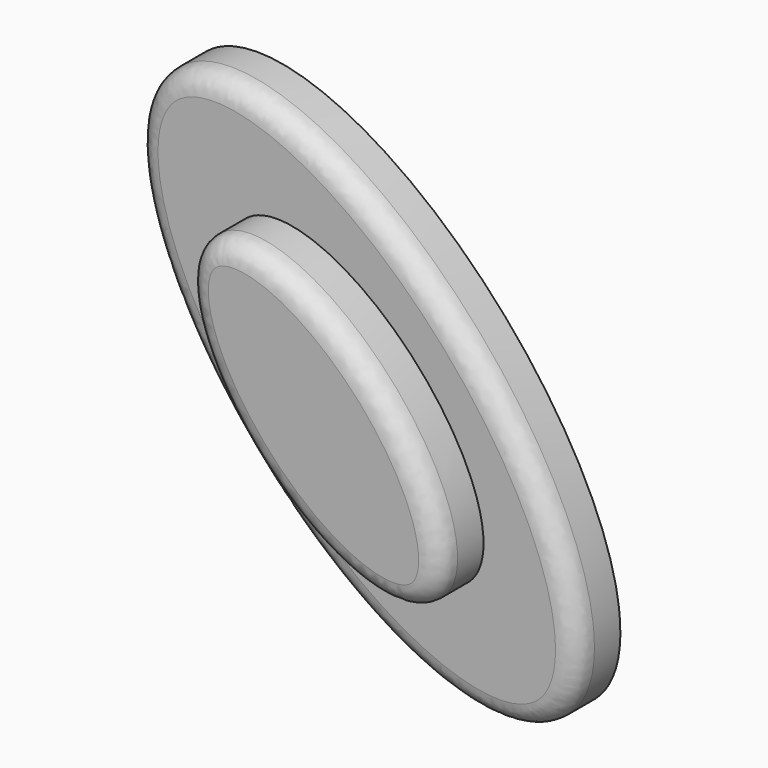
from build123d import *

# Parameters (mm, degrees)
F1_DEPTH = 12.7
F3_DEPTH = 12.7
F4_R     = 5.08


with BuildPart() as f1:
    # F0 (on Front) → F1 (new body)
    with BuildSketch(Plane.XZ):
        with BuildLine():
            add(Edge.make_bspline(
                [(45.9132567048, -51.8883131444), (87.3111627168, -15.2574694999), (-2.2576753464, 44.2595783945), (-91.8265134096, 103.7766262889), (-43.6555813584, 7.62873475), (4.5153506928, -88.519156789), (45.9132567048, -51.8883131444)],
                knots=[0, 0, 0, 2.0943951024, 2.0943951024, 4.1887902048, 4.1887902048, 6.2831853072, 6.2831853072, 6.2831853072], degree=2, weights=[1, 0.5, 1, 0.5, 1, 0.5, 1]))
        make_face()
    extrude(amount=-F1_DEPTH)

    # F2 (on face) → F3 (join)
    with BuildSketch(Plane.XZ):
        with BuildLine():
            add(Edge.make_bspline(
                [(-26.4271013439, 28.8640391082), (-50.1823996848, 7.1143569394), (1.3359015015, -25.3068606385), (52.8542026877, -57.7280782163), (25.0911998424, -3.5571784697), (-2.671803003, 50.6137212769), (-26.4271013439, 28.8640391082)],
                knots=[0, 0, 0, 2.0943951024, 2.0943951024, 4.1887902048, 4.1887902048, 6.2831853072, 6.2831853072, 6.2831853072], degree=2, weights=[1, 0.5, 1, 0.5, 1, 0.5, 1]))
        make_face()
    extrude(amount=F3_DEPTH)

    # F4
    f4_edges = [f1.edges().sort_by_distance(p)[0] for p in [
        (-45.91324, 0, 51.888328),
        (26.427095, -12.7, -28.864045),
    ]]
    fillet(f4_edges, radius=F4_R)


solid = f1.part
